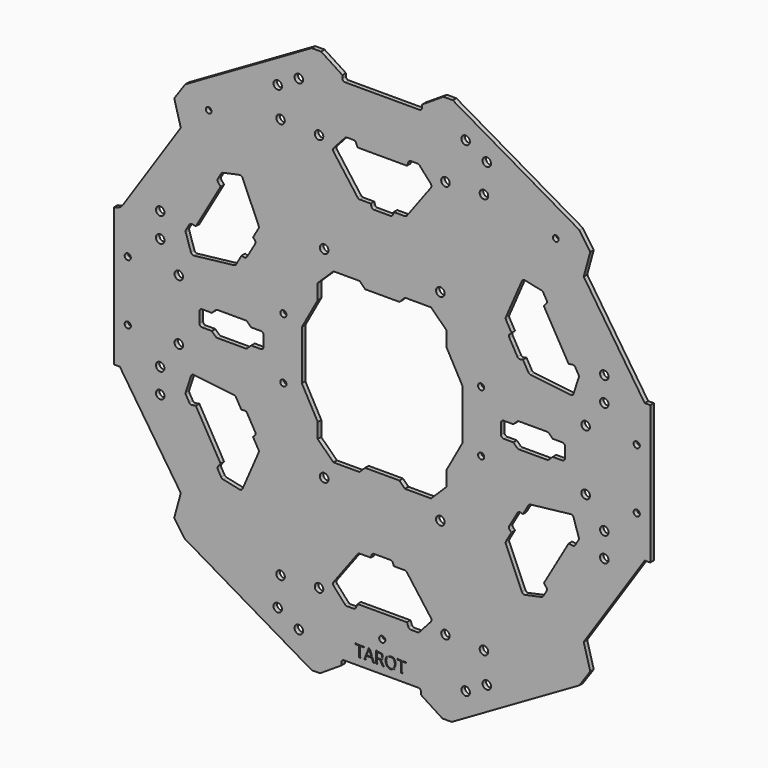
from build123d import *

# Parameters (mm, degrees)
F1_DEPTH      = 1.6
F3_DEPTH      = 25
F5_ANGLE      = 30
F7_DEPTH      = 25
F9_R          = 1
F10_T1_DEPTH  = 1.6
F8_R          = 1.575
F8_R_2        = 1.125
F8_R_3        = 1.55
F8_R_4        = 1.05
F11_DEPTH     = 25
F12_R         = 1.125
F12_R_2       = 1.55
F13_DEPTH     = 25
F14_TEXT_SIZE = 5.9027777778
F15_DEPTH     = 0.3
F17_DEPTH     = 25
F19_DEPTH     = 25


# Not quite as in the source:
# - a fillet or chamfer that OpenCascade refuses, or shapes differently, is made with other operations: its cross-section is extruded or revolved along the edge and cut away or added
# - a feature names something its author has since deleted; it is built from what else it names
# - Text() gives the source's letters only with a copy of the font that has no kerning and outlines rounded to 1/6400 em; it was checked with that copy


with BuildPart() as f1:
    # F0 (on Front) → F1 (new body)
    with BuildSketch(Plane.XZ):
        Polygon((57.1576766498, 99), (-55.4256258422, 99), (-113.2374158301, -1.1329575356), (-57.5965023401, -99), (55.4256258422, -99), (113.4493278958, 1.5), align=None)
    extrude(amount=F1_DEPTH)

    # F2 (on face) → F3 (cut)
    with BuildSketch(Plane.XZ.offset(1.6)):
        Polygon((-71.8315208362, 70.5841563268), (-70.0841444893, 69.5753081226), (-34.2213739477, 87.291450171), (-31.9495553203, 96), (-25.625, 99), (-33.125, 99), (-55.4256258422, 99), align=None)
        Polygon((-95.2960565549, 25.9069954689), (-97.0434329018, 26.9158436732), (-113.2374158301, -1.1329575356), (-98.5810343261, -26.9121301096), (-99.1132164235, -20.330873453), (-92.7073003551, -14.0091458944), align=None)
        Polygon((31.9495553203, -96), (25.625, -99), (33.125, -99), (55.4256258422, -99), (71.8315208362, -70.5841563268), (70.0841444893, -69.5753081226), (34.2213739477, -87.291450171), align=None)
        Polygon((102.2990149747, 20.8129084996), (98.5490149747, 27.308099028), (99.1132164235, 20.330873453), (92.7073003551, 14.0091458944), (95.2960565549, -25.9069954689), (97.0434329018, -26.9158436732), (113.4493278958, 1.5), align=None)
    extrude(amount=-F3_DEPTH, mode=Mode.SUBTRACT)


with BuildPart() as f1_1:
    # F5: moved
    add(f1.part.rotate(Axis((0, -26.3710785657, 0), (0, -1, 0)), F5_ANGLE))

    # F6 (on face) → F7 (cut)
    with BuildSketch(Plane.XZ.offset(1.6)):
        Polygon((-14.5, 92.5), (0, 92.5), (14.5, 92.5), (14.5, 94.5), (22.25, 99.5), (25.6609446469, 99.5), (0, 114.3153532995), (-25.6609446469, 99.5), (-22.25, 99.5), (-14.5, 94.5), align=None)
        Polygon((14.1199658044, -92.7194128451), (-0.3800341956, -92.7194128451), (-14.8800341956, -92.7194128451), (-14.8800341956, -94.7194128451), (-22.6300341956, -99.7194128451), (-26.0409788425, -99.7194128451), (-0.3800341956, -114.5347661447), (25.2809104513, -99.7194128451), (21.8699658044, -99.7194128451), (14.1199658044, -94.7194128451), align=None)
    extrude(amount=-F7_DEPTH, mode=Mode.SUBTRACT)

    # F9
    f9_edges = [f1_1.edges().sort_by_distance(p)[0] for p in [
        (-14.5, -0.8, 92.5),
        (14.5, -0.8, 92.5),
        (-14.880034, -0.8, -92.719413),
        (14.119966, -0.8, -92.719413),
    ]]
    fillet(f9_edges, radius=F9_R)

    # F10: fillet of radius 4 on 1 edges, made by hand

    # F10_s2 → F10_t1 (join)
    with BuildSketch(Plane.XZ):
        with BuildLine():
            ThreePointArc((-97.5, 25.2119120656), (-95.6824068095, 25.712492863), (-94.2959800526, 26.9900088074))
            Line((-94.2959800526, 26.9900088074), (-95.4823035915, 25.2119120656))
            Line((-95.4823035915, 25.2119120656), (-97.5, 25.2119120656))
        make_face()
    extrude(amount=F10_T1_DEPTH)

    # F8 (on face) → F11 (cut)
    with BuildSketch(Plane.XZ.offset(1.6)):
        with Locations((-21.125, 36.625)):
            Circle(F8_R)
        with Locations((21.125, 36.625)):
            Circle(F8_R)
        with Locations((-21.125, -36.625)):
            Circle(F8_R)
        with Locations((21.125, -36.625)):
            Circle(F8_R)
        with Locations((-35.975, 11.1)):
            Circle(F8_R_2)
        with Locations((-35.975, -11.1)):
            Circle(F8_R_2)
        with Locations((35.975, 11.1)):
            Circle(F8_R_2)
        with Locations((35.975, -11.1)):
            Circle(F8_R_2)
        with Locations((-23, 72.5)):
            Circle(F8_R_3)
        with Locations((23, 72.5)):
            Circle(F8_R_3)
        with Locations((23, -72.5)):
            Circle(F8_R_3)
        with Locations((-23, -72.5)):
            Circle(F8_R_3)
        with Locations((-37, 73)):
            Circle(F8_R_3)
        with Locations((37, 73)):
            Circle(F8_R_3)
        with Locations((-37, -73)):
            Circle(F8_R_3)
        with Locations((37, -73)):
            Circle(F8_R_3)
        with Locations((0, -81.4694128451)):
            Circle(F8_R_2)
        with Locations((-63.15, 67.4056439279)):
            Circle(F8_R_4)
        with Locations((63.15, 67.4056439279)):
            Circle(F8_R_4)
    extrude(amount=-F11_DEPTH, mode=Mode.SUBTRACT)

    # F12 (on face) → F13 (cut)
    with BuildSketch(Plane.XZ.offset(1.6)):
        with Locations((-92.575, -10.925)):
            Circle(F12_R)
        with Locations((-92.575, 10.925)):
            Circle(F12_R)
        with Locations((92.575, -10.925)):
            Circle(F12_R)
        with Locations((92.575, 10.925)):
            Circle(F12_R)
        with Locations((-74, 11)):
            Circle(F12_R_2)
        with Locations((-74, -11)):
            Circle(F12_R_2)
        with Locations((74, 11)):
            Circle(F12_R_2)
        with Locations((74, -11)):
            Circle(F12_R_2)
        with Locations((-80.7805959792, -20.4734375053)):
            Circle(F12_R_2)
        with Locations((-80.7805959792, -29.3734375053)):
            Circle(F12_R_2)
        with Locations((-80.7805959792, 20.4734375053)):
            Circle(F12_R_2)
        with Locations((-80.7805959792, 29.3734375053)):
            Circle(F12_R_2)
        with Locations((80.7805959792, -20.4734375053)):
            Circle(F12_R_2)
        with Locations((80.7805959792, -29.3734375053)):
            Circle(F12_R_2)
        with Locations((80.7805959792, 29.3734375053)):
            Circle(F12_R_2)
        with Locations((80.7805959792, 20.4734375053)):
            Circle(F12_R_2)
        with Locations((-30.35, -88.2136832429)):
            Circle(F12_R_2)
        with Locations((-38.0279258959, -83.712632928)):
            Circle(F12_R_2)
        with Locations((38.0279258959, -83.712632928)):
            Circle(F12_R_2)
        with Locations((30.35, -88.2136832429)):
            Circle(F12_R_2)
        with Locations((-30.35, 88.2136832429)):
            Circle(F12_R_2)
        with Locations((30.35, 88.2136832429)):
            Circle(F12_R_2)
        with Locations((-38.0279258959, 83.712632928)):
            Circle(F12_R_2)
        with Locations((38.0279258959, 83.712632928)):
            Circle(F12_R_2)
    extrude(amount=-F13_DEPTH, mode=Mode.SUBTRACT)

    # F14 (on face) → F15 (cut)
    with BuildSketch(Plane.XZ.offset(1.6)):
        with Locations((-9.8000374508, -90.011609748)):
            Text('TAROT', F14_TEXT_SIZE, font='Open Sans', text_align=(TextAlign.LEFT, TextAlign.BOTTOM))
    extrude(amount=-F15_DEPTH, mode=Mode.SUBTRACT)

    # F16 (on face) → F17 (cut)
    with BuildSketch(Plane.XZ.offset(1.6)):
        Polygon((-23.4631427428, 19.5), (-29.25, 9), (-29.25, 0), (-29.25, -9), (-23.4631427428, -19.5), (-23.4631427428, -25), (-17.75, -30.6), (-8.25, -30.6), (-6.25, -28.6), (0, -28.6), (6.25, -28.6), (8.25, -30.6), (17.75, -30.6), (23.4631427428, -25), (23.4631427428, -19.5), (29.25, -9), (29.25, 0), (29.25, 9), (23.4631427428, 19.5), (23.4631427428, 25), (17.75, 30.6), (8.25, 30.6), (6.25, 28.6), (0, 28.6), (-6.25, 28.6), (-8.25, 30.6), (-17.75, 30.6), (-23.4631427428, 25), align=None)
        with BuildLine():
            Line((9, 73.1), (0, 73.1))
            Line((0, 73.1), (-9, 73.1))
            Line((-9, 73.1), (-9.5052474863, 74.4098776309))
            ThreePointArc((-9.5052474863, 74.4098776309), (-9.8725074966, 74.8745840257), (-10.438246999, 75.05))
            Line((-10.438246999, 75.05), (-12.806663998, 75.05))
            ThreePointArc((-12.806663998, 75.05), (-13.2136015301, 74.9634559896), (-13.5501030501, 74.71880369))
            Line((-13.5501030501, 74.71880369), (-17.6531240514, 70.1579047453))
            ThreePointArc((-17.6531240514, 70.1579047453), (-17.9085730801, 69.5362455355), (-17.7128099993, 68.8932904861))
            Line((-17.7128099993, 68.8932904861), (-8.9668850061, 57.1041894308))
            ThreePointArc((-8.9668850061, 57.1041894308), (-8.6133094644, 56.806744558), (-8.1637600061, 56.7))
            Line((-8.1637600061, 56.7), (-4.1670308927, 56.7))
            Line((-4.1670308927, 56.7), (-3.9449051726, 55.8477821946))
            ThreePointArc((-3.9449051726, 55.8477821946), (-3.588701032, 55.3087295641), (-2.9772346819, 55.1))
            Line((-2.9772346819, 55.1), (0, 55.1))
            Line((0, 55.1), (2.9772346819, 55.1))
            ThreePointArc((2.9772346819, 55.1), (3.588701032, 55.3087295641), (3.9449051726, 55.8477821946))
            Line((3.9449051726, 55.8477821946), (4.1670308927, 56.7))
            Line((4.1670308927, 56.7), (8.1637600061, 56.7))
            ThreePointArc((8.1637600061, 56.7), (8.6133094644, 56.806744558), (8.9668850061, 57.1041894308))
            Line((8.9668850061, 57.1041894308), (17.7128099993, 68.8932904861))
            ThreePointArc((17.7128099993, 68.8932904861), (17.9085730801, 69.5362455355), (17.6531240514, 70.1579047453))
            Line((17.6531240514, 70.1579047453), (13.5501030501, 74.71880369))
            ThreePointArc((13.5501030501, 74.71880369), (13.2136015301, 74.9634559896), (12.806663998, 75.05))
            Line((12.806663998, 75.05), (10.438246999, 75.05))
            ThreePointArc((10.438246999, 75.05), (9.8725074966, 74.8745840257), (9.5052474863, 74.4098776309))
            Line((9.5052474863, 74.4098776309), (9, 73.1))
        make_face()
        with BuildLine():
            ThreePointArc((-69.5850898114, 19.7908984879), (-69.1744416576, 19.2588435348), (-68.5197447109, 19.1069018112))
            Line((-68.5197447109, 19.1069018112), (-53.9371212127, 20.7865445073))
            ThreePointArc((-53.9371212127, 20.7865445073), (-53.5027386257, 20.9440274722), (-53.1855203976, 21.2799764443))
            Line((-53.1855203976, 21.2799764443), (-51.1871558409, 24.7412453885))
            Line((-51.1871558409, 24.7412453885), (-50.3380507119, 24.5075030023))
            ThreePointArc((-50.3380507119, 24.5075030023), (-49.6931153696, 24.5464585218), (-49.2066170895, 24.9716391325))
            Line((-49.2066170895, 24.9716391325), (-47.7179997485, 27.55))
            Line((-47.7179997485, 27.55), (-46.2293824076, 30.1283608675))
            ThreePointArc((-46.2293824076, 30.1283608675), (-46.1044143376, 30.7622710423), (-46.3931455392, 31.3402791923))
            Line((-46.3931455392, 31.3402791923), (-47.0201249482, 31.9587546115))
            Line((-47.0201249482, 31.9587546115), (-45.0217603915, 35.4200235557))
            ThreePointArc((-45.0217603915, 35.4200235557), (-44.8894291614, 35.8627170858), (-44.9702362065, 36.3176449235))
            Line((-44.9702362065, 36.3176449235), (-50.8069347116, 49.7863886748))
            ThreePointArc((-50.8069347116, 49.7863886748), (-51.2658685775, 50.2774020007), (-51.93196576, 50.3670062573))
            Line((-51.93196576, 50.3670062573), (-57.9333306109, 49.0941353103))
            ThreePointArc((-57.9333306109, 49.0941353103), (-58.3134564775, 48.9250425953), (-58.591874555, 48.61589636))
            Line((-58.591874555, 48.61589636), (-59.7760830545, 46.5647870721))
            ThreePointArc((-59.7760830545, 46.5647870721), (-59.9070381157, 45.987134304), (-59.6882205777, 45.4367246078))
            Line((-59.6882205777, 45.4367246078), (-58.8064570166, 44.3442286341))
            Line((-58.8064570166, 44.3442286341), (-63.3064570166, 36.55))
            Line((-63.3064570166, 36.55), (-67.8064570166, 28.7557713659))
            Line((-67.8064570166, 28.7557713659), (-69.193468064, 28.9731530231))
            ThreePointArc((-69.193468064, 28.9731530231), (-69.7795456124, 28.8874497217), (-70.2143300535, 28.4852129279))
            Line((-70.2143300535, 28.4852129279), (-71.398538553, 26.43410364))
            ThreePointArc((-71.398538553, 26.43410364), (-71.5270580075, 26.0384133943), (-71.483433661, 25.6246683797))
            Line((-71.483433661, 25.6246683797), (-69.5850898114, 19.7908984879))
        make_face()
        with BuildLine():
            ThreePointArc((-51.93196576, -50.3670062573), (-51.2658685775, -50.2774020007), (-50.8069347116, -49.7863886748))
            Line((-50.8069347116, -49.7863886748), (-44.9702362065, -36.3176449235))
            ThreePointArc((-44.9702362065, -36.3176449235), (-44.8894291614, -35.8627170858), (-45.0217603915, -35.4200235557))
            Line((-45.0217603915, -35.4200235557), (-47.0201249482, -31.9587546115))
            Line((-47.0201249482, -31.9587546115), (-46.3931455392, -31.3402791923))
            ThreePointArc((-46.3931455392, -31.3402791923), (-46.1044143376, -30.7622710423), (-46.2293824076, -30.1283608675))
            Line((-46.2293824076, -30.1283608675), (-47.7179997485, -27.55))
            Line((-47.7179997485, -27.55), (-49.2066170895, -24.9716391325))
            ThreePointArc((-49.2066170895, -24.9716391325), (-49.6931153696, -24.5464585218), (-50.3380507119, -24.5075030023))
            Line((-50.3380507119, -24.5075030023), (-51.1871558409, -24.7412453885))
            Line((-51.1871558409, -24.7412453885), (-53.1855203976, -21.2799764443))
            ThreePointArc((-53.1855203976, -21.2799764443), (-53.5027386257, -20.9440274722), (-53.9371212127, -20.7865445073))
            Line((-53.9371212127, -20.7865445073), (-68.5197447109, -19.1069018112))
            ThreePointArc((-68.5197447109, -19.1069018112), (-69.1744416576, -19.2588435348), (-69.5850898114, -19.7908984879))
            Line((-69.5850898114, -19.7908984879), (-71.483433661, -25.6246683797))
            ThreePointArc((-71.483433661, -25.6246683797), (-71.5270580075, -26.0384133943), (-71.398538553, -26.43410364))
            Line((-71.398538553, -26.43410364), (-70.2143300535, -28.4852129279))
            ThreePointArc((-70.2143300535, -28.4852129279), (-69.7795456124, -28.8874497217), (-69.193468064, -28.9731530231))
            Line((-69.193468064, -28.9731530231), (-67.8064570166, -28.7557713659))
            Line((-67.8064570166, -28.7557713659), (-63.3064570166, -36.55))
            Line((-63.3064570166, -36.55), (-58.8064570166, -44.3442286341))
            Line((-58.8064570166, -44.3442286341), (-59.6882205777, -45.4367246078))
            ThreePointArc((-59.6882205777, -45.4367246078), (-59.9070381157, -45.987134304), (-59.7760830545, -46.5647870721))
            Line((-59.7760830545, -46.5647870721), (-58.591874555, -48.61589636))
            ThreePointArc((-58.591874555, -48.61589636), (-58.3134564775, -48.9250425953), (-57.9333306109, -49.0941353103))
            Line((-57.9333306109, -49.0941353103), (-51.93196576, -50.3670062573))
        make_face()
        with BuildLine():
            ThreePointArc((17.6531240514, -70.1579047453), (17.9085730801, -69.5362455355), (17.7128099993, -68.8932904861))
            Line((17.7128099993, -68.8932904861), (8.9668850061, -57.1041894308))
            ThreePointArc((8.9668850061, -57.1041894308), (8.6133094644, -56.806744558), (8.1637600061, -56.7))
            Line((8.1637600061, -56.7), (4.1670308927, -56.7))
            Line((4.1670308927, -56.7), (3.9449051726, -55.8477821946))
            ThreePointArc((3.9449051726, -55.8477821946), (3.588701032, -55.3087295641), (2.9772346819, -55.1))
            Line((2.9772346819, -55.1), (0, -55.1))
            Line((0, -55.1), (-2.9772346819, -55.1))
            ThreePointArc((-2.9772346819, -55.1), (-3.588701032, -55.3087295641), (-3.9449051726, -55.8477821946))
            Line((-3.9449051726, -55.8477821946), (-4.1670308927, -56.7))
            Line((-4.1670308927, -56.7), (-8.1637600061, -56.7))
            ThreePointArc((-8.1637600061, -56.7), (-8.6133094644, -56.806744558), (-8.9668850061, -57.1041894308))
            Line((-8.9668850061, -57.1041894308), (-17.7128099993, -68.8932904861))
            ThreePointArc((-17.7128099993, -68.8932904861), (-17.9085730801, -69.5362455355), (-17.6531240514, -70.1579047453))
            Line((-17.6531240514, -70.1579047453), (-13.5501030501, -74.71880369))
            ThreePointArc((-13.5501030501, -74.71880369), (-13.2136015301, -74.9634559896), (-12.806663998, -75.05))
            Line((-12.806663998, -75.05), (-10.438246999, -75.05))
            ThreePointArc((-10.438246999, -75.05), (-9.8725074966, -74.8745840257), (-9.5052474863, -74.4098776309))
            Line((-9.5052474863, -74.4098776309), (-9, -73.1))
            Line((-9, -73.1), (0, -73.1))
            Line((0, -73.1), (9, -73.1))
            Line((9, -73.1), (9.5052474863, -74.4098776309))
            ThreePointArc((9.5052474863, -74.4098776309), (9.8725074966, -74.8745840257), (10.438246999, -75.05))
            Line((10.438246999, -75.05), (12.806663998, -75.05))
            ThreePointArc((12.806663998, -75.05), (13.2136015301, -74.9634559896), (13.5501030501, -74.71880369))
            Line((13.5501030501, -74.71880369), (17.6531240514, -70.1579047453))
        make_face()
        with BuildLine():
            ThreePointArc((69.5850898114, -19.7908984879), (69.1744416576, -19.2588435348), (68.5197447109, -19.1069018112))
            Line((68.5197447109, -19.1069018112), (53.9371212127, -20.7865445073))
            ThreePointArc((53.9371212127, -20.7865445073), (53.5027386257, -20.9440274722), (53.1855203976, -21.2799764443))
            Line((53.1855203976, -21.2799764443), (51.1871558409, -24.7412453885))
            Line((51.1871558409, -24.7412453885), (50.3380507119, -24.5075030023))
            ThreePointArc((50.3380507119, -24.5075030023), (49.6931153696, -24.5464585218), (49.2066170895, -24.9716391325))
            Line((49.2066170895, -24.9716391325), (47.7179997485, -27.55))
            Line((47.7179997485, -27.55), (46.2293824076, -30.1283608675))
            ThreePointArc((46.2293824076, -30.1283608675), (46.1044143376, -30.7622710423), (46.3931455392, -31.3402791923))
            Line((46.3931455392, -31.3402791923), (47.0201249482, -31.9587546115))
            Line((47.0201249482, -31.9587546115), (45.0217603915, -35.4200235557))
            ThreePointArc((45.0217603915, -35.4200235557), (44.8894291614, -35.8627170858), (44.9702362065, -36.3176449235))
            Line((44.9702362065, -36.3176449235), (50.8069347116, -49.7863886748))
            ThreePointArc((50.8069347116, -49.7863886748), (51.2658685775, -50.2774020007), (51.93196576, -50.3670062573))
            Line((51.93196576, -50.3670062573), (57.9333306109, -49.0941353103))
            ThreePointArc((57.9333306109, -49.0941353103), (58.3134564775, -48.9250425953), (58.591874555, -48.61589636))
            Line((58.591874555, -48.61589636), (59.7760830545, -46.5647870721))
            ThreePointArc((59.7760830545, -46.5647870721), (59.9070381157, -45.987134304), (59.6882205777, -45.4367246078))
            Line((59.6882205777, -45.4367246078), (58.8064570166, -44.3442286341))
            Line((58.8064570166, -44.3442286341), (63.3064570166, -36.55))
            Line((63.3064570166, -36.55), (67.8064570166, -28.7557713659))
            Line((67.8064570166, -28.7557713659), (69.193468064, -28.9731530231))
            ThreePointArc((69.193468064, -28.9731530231), (69.7795456124, -28.8874497217), (70.2143300535, -28.4852129279))
            Line((70.2143300535, -28.4852129279), (71.398538553, -26.43410364))
            ThreePointArc((71.398538553, -26.43410364), (71.5270580075, -26.0384133943), (71.483433661, -25.6246683797))
            Line((71.483433661, -25.6246683797), (69.5850898114, -19.7908984879))
        make_face()
        with BuildLine():
            ThreePointArc((51.93196576, 50.3670062573), (51.2658685775, 50.2774020007), (50.8069347116, 49.7863886748))
            Line((50.8069347116, 49.7863886748), (44.9702362065, 36.3176449235))
            ThreePointArc((44.9702362065, 36.3176449235), (44.8894291614, 35.8627170858), (45.0217603915, 35.4200235557))
            Line((45.0217603915, 35.4200235557), (47.0201249482, 31.9587546115))
            Line((47.0201249482, 31.9587546115), (46.3931455392, 31.3402791923))
            ThreePointArc((46.3931455392, 31.3402791923), (46.1044143376, 30.7622710423), (46.2293824076, 30.1283608675))
            Line((46.2293824076, 30.1283608675), (47.7179997485, 27.55))
            Line((47.7179997485, 27.55), (49.2066170895, 24.9716391325))
            ThreePointArc((49.2066170895, 24.9716391325), (49.6931153696, 24.5464585218), (50.3380507119, 24.5075030023))
            Line((50.3380507119, 24.5075030023), (51.1871558409, 24.7412453885))
            Line((51.1871558409, 24.7412453885), (53.1855203976, 21.2799764443))
            ThreePointArc((53.1855203976, 21.2799764443), (53.5027386257, 20.9440274722), (53.9371212127, 20.7865445073))
            Line((53.9371212127, 20.7865445073), (68.5197447109, 19.1069018112))
            ThreePointArc((68.5197447109, 19.1069018112), (69.1744416576, 19.2588435348), (69.5850898114, 19.7908984879))
            Line((69.5850898114, 19.7908984879), (71.483433661, 25.6246683797))
            ThreePointArc((71.483433661, 25.6246683797), (71.5270580075, 26.0384133943), (71.398538553, 26.43410364))
            Line((71.398538553, 26.43410364), (70.2143300535, 28.4852129279))
            ThreePointArc((70.2143300535, 28.4852129279), (69.7795456124, 28.8874497217), (69.193468064, 28.9731530231))
            Line((69.193468064, 28.9731530231), (67.8064570166, 28.7557713659))
            Line((67.8064570166, 28.7557713659), (63.3064570166, 36.55))
            Line((63.3064570166, 36.55), (58.8064570166, 44.3442286341))
            Line((58.8064570166, 44.3442286341), (59.6882205777, 45.4367246078))
            ThreePointArc((59.6882205777, 45.4367246078), (59.9070381157, 45.987134304), (59.7760830545, 46.5647870721))
            Line((59.7760830545, 46.5647870721), (58.591874555, 48.61589636))
            ThreePointArc((58.591874555, 48.61589636), (58.3134564775, 48.9250425953), (57.9333306109, 49.0941353103))
            Line((57.9333306109, 49.0941353103), (51.93196576, 50.3670062573))
        make_face()
    extrude(amount=-F17_DEPTH, mode=Mode.SUBTRACT)

    # F18 (on face) → F19 (cut)
    with BuildSketch(Plane.XZ.offset(1.6)):
        with BuildLine():
            Line((-66.5, 1.9), (-66.5, 0))
            Line((-66.5, 0), (-66.5, -1.9))
            ThreePointArc((-66.5, -1.9), (-66.2071067812, -2.6071067812), (-65.5, -2.9))
            Line((-65.5, -2.9), (-62, -2.9))
            Line((-62, -2.9), (-60.6409152193, -4.2179003935))
            ThreePointArc((-60.6409152193, -4.2179003935), (-60.3203353604, -4.4267956607), (-59.9447693832, -4.5))
            Line((-59.9447693832, -4.5), (-54.85, -4.5))
            Line((-54.85, -4.5), (-49.7552306168, -4.5))
            ThreePointArc((-49.7552306168, -4.5), (-49.3796646396, -4.4267956607), (-49.0590847807, -4.2179003935))
            Line((-49.0590847807, -4.2179003935), (-47.7, -2.9))
            Line((-47.7, -2.9), (-44.2, -2.9))
            ThreePointArc((-44.2, -2.9), (-43.4928932188, -2.6071067812), (-43.2, -1.9))
            Line((-43.2, -1.9), (-43.2, 0))
            Line((-43.2, 0), (-43.2, 1.9))
            ThreePointArc((-43.2, 1.9), (-43.4928932188, 2.6071067812), (-44.2, 2.9))
            Line((-44.2, 2.9), (-47.7, 2.9))
            Line((-47.7, 2.9), (-49.0590847807, 4.2179003935))
            ThreePointArc((-49.0590847807, 4.2179003935), (-49.3796646396, 4.4267956607), (-49.7552306168, 4.5))
            Line((-49.7552306168, 4.5), (-54.85, 4.5))
            Line((-54.85, 4.5), (-59.9447693832, 4.5))
            ThreePointArc((-59.9447693832, 4.5), (-60.3203353604, 4.4267956607), (-60.6409152193, 4.2179003935))
            Line((-60.6409152193, 4.2179003935), (-62, 2.9))
            Line((-62, 2.9), (-65.5, 2.9))
            ThreePointArc((-65.5, 2.9), (-66.2071067812, 2.6071067812), (-66.5, 1.9))
        make_face()
        with BuildLine():
            Line((60.6409152193, -4.2179003935), (62, -2.9))
            Line((62, -2.9), (65.5, -2.9))
            ThreePointArc((65.5, -2.9), (66.2071067812, -2.6071067812), (66.5, -1.9))
            Line((66.5, -1.9), (66.5, 0))
            Line((66.5, 0), (66.5, 1.9))
            ThreePointArc((66.5, 1.9), (66.2071067812, 2.6071067812), (65.5, 2.9))
            Line((65.5, 2.9), (62, 2.9))
            Line((62, 2.9), (60.6409152193, 4.2179003935))
            ThreePointArc((60.6409152193, 4.2179003935), (60.3203353604, 4.4267956607), (59.9447693832, 4.5))
            Line((59.9447693832, 4.5), (54.85, 4.5))
            Line((54.85, 4.5), (49.7552306168, 4.5))
            ThreePointArc((49.7552306168, 4.5), (49.3796646396, 4.4267956607), (49.0590847807, 4.2179003935))
            Line((49.0590847807, 4.2179003935), (47.7, 2.9))
            Line((47.7, 2.9), (44.2, 2.9))
            ThreePointArc((44.2, 2.9), (43.4928932188, 2.6071067812), (43.2, 1.9))
            Line((43.2, 1.9), (43.2, 0))
            Line((43.2, 0), (43.2, -1.9))
            ThreePointArc((43.2, -1.9), (43.4928932188, -2.6071067812), (44.2, -2.9))
            Line((44.2, -2.9), (47.7, -2.9))
            Line((47.7, -2.9), (49.0590847807, -4.2179003935))
            ThreePointArc((49.0590847807, -4.2179003935), (49.3796646396, -4.4267956607), (49.7552306168, -4.5))
            Line((49.7552306168, -4.5), (54.85, -4.5))
            Line((54.85, -4.5), (59.9447693832, -4.5))
            ThreePointArc((59.9447693832, -4.5), (60.3203353604, -4.4267956607), (60.6409152193, -4.2179003935))
        make_face()
    extrude(amount=-F19_DEPTH, mode=Mode.SUBTRACT)


solid = f1_1.part
